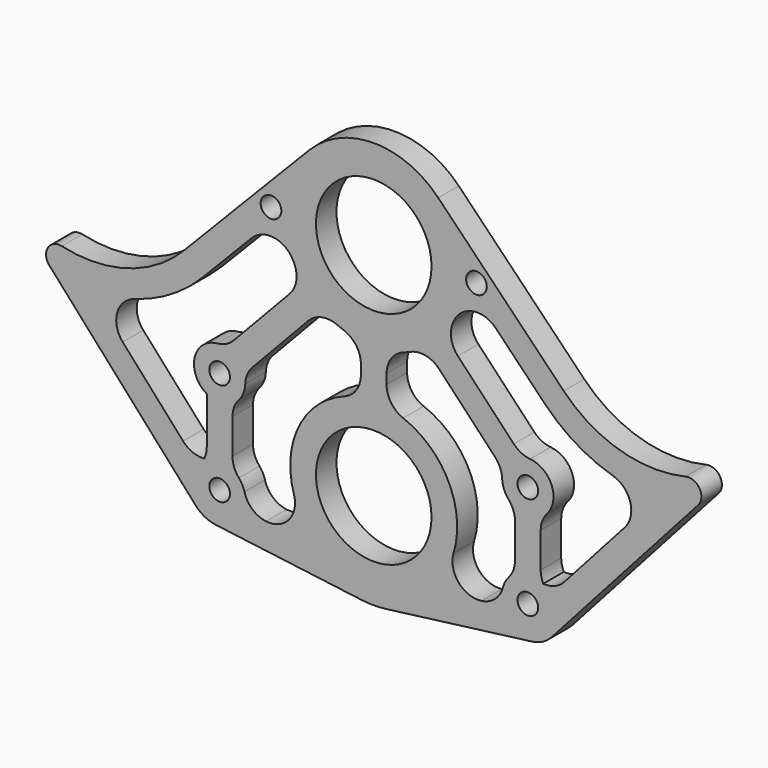
from build123d import *

# Parameters (mm, degrees)
F0_R        = 2.5527
F0_R_2      = 14.2875
F1_DEPTH    = 6.35
F3_DEPTH    = 25.4
F4_T1_DEPTH = 6.35


# Not quite as in the source:
# - a fillet or chamfer that OpenCascade refuses, or shapes differently, is made with other operations: its cross-section is extruded or revolved along the edge and cut away or added


with BuildPart() as f1:
    # F0 (on Front) → F1 (new body)
    with BuildSketch(Plane.XZ):
        with BuildLine():
            ThreePointArc((-3.0331353108, -25.2060360773), (0, -25.4), (3.0331353108, -25.2060360773))
            Line((3.0331353108, -25.2060360773), (39.1110451036, -20.5728453591))
            ThreePointArc((39.1110451036, -20.5728453591), (41.7972497423, -19.7238344651), (44.0177169487, -17.9900408661))
            Line((44.0177169487, -17.9900408661), (80.2059498117, 22.4920129361))
            ThreePointArc((80.2059498117, 22.4920129361), (80.5691803237, 26.2285207166), (77.1152341344, 27.6994668475))
            ThreePointArc((77.1152341344, 27.6994668475), (60.8820938076, 28.1479627769), (46.9763621139, 36.5352519414))
            Line((46.9763621139, 36.5352519414), (15.9477554983, 68.5021550209))
            ThreePointArc((15.9477554983, 68.5021550209), (0, 75.2475), (-15.9477554983, 68.5021550209))
            Line((-15.9477554983, 68.5021550209), (-46.9763621139, 36.5352519414))
            ThreePointArc((-46.9763621139, 36.5352519414), (-60.8820938076, 28.1479627769), (-77.1152341344, 27.6994668475))
            ThreePointArc((-77.1152341344, 27.6994668475), (-80.5691803237, 26.2285207166), (-80.2059498117, 22.4920129361))
            Line((-80.2059498117, 22.4920129361), (-44.0177169487, -17.9900408661))
            ThreePointArc((-44.0177169487, -17.9900408661), (-41.7972497423, -19.7238344651), (-39.1110451036, -20.5728453591))
            Line((-39.1110451036, -20.5728453591), (-3.0331353108, -25.2060360773))
        make_face()
        with Locations((-38.1, -12.7)):
            Circle(F0_R, mode=Mode.SUBTRACT)
        with Locations((0, -1.5875)):
            Circle(F0_R_2, mode=Mode.SUBTRACT)
        with Locations((-38.1, 12.7)):
            Circle(F0_R, mode=Mode.SUBTRACT)
        with Locations((38.1, -12.7)):
            Circle(F0_R, mode=Mode.SUBTRACT)
        with Locations((38.1, 12.7)):
            Circle(F0_R, mode=Mode.SUBTRACT)
        with Locations((-25.4, 53.0225)):
            Circle(F0_R, mode=Mode.SUBTRACT)
        with Locations((0, 53.0225)):
            Circle(F0_R_2, mode=Mode.SUBTRACT)
        with Locations((25.4, 53.0225)):
            Circle(F0_R, mode=Mode.SUBTRACT)
    extrude(amount=F1_DEPTH)

    # F2 (on face) → F3 (cut)
    with BuildSketch(Plane.XZ.offset(6.35)):
        with BuildLine():
            ThreePointArc((-43.3811914248, -9.1741643352), (-42.441704222, -8.0661997833), (-41.275, -7.200738686))
            Line((-41.275, -7.200738686), (-41.275, 7.200738686))
            ThreePointArc((-41.275, 7.200738686), (-44.0004697722, 15.046690535), (-36.6309164423, 18.8777255929))
            Line((-36.6309164423, 18.8777255929), (-17.4151480361, 39.2144138227))
            ThreePointArc((-17.4151480361, 39.2144138227), (-20.0010259245, 43.331804103), (-21.6296875, 47.9129752029))
            ThreePointArc((-21.6296875, 47.9129752029), (-24.6257359251, 46.7198802953), (-27.8214787465, 47.1523261797))
            Line((-27.8214787465, 47.1523261797), (-42.4198605429, 32.112493364))
            ThreePointArc((-42.4198605429, 32.112493364), (-54.9895844041, 23.5171709652), (-69.9173374643, 20.510559308))
            Line((-69.9173374643, 20.510559308), (-43.3811914248, -9.1741643352))
        make_face()
        with BuildLine():
            Line((-34.925, 7.200738686), (-34.925, -7.200738686))
            ThreePointArc((-34.925, -7.200738686), (-32.0996562634, -10.6219299715), (-32.2039292281, -15.0577212415))
            Line((-32.2039292281, -15.0577212415), (-13.1332337576, -17.5068145995))
            ThreePointArc((-13.1332337576, -17.5068145995), (-19.9026130173, 3.870741597), (-3.175, 18.8043067186))
            Line((-3.175, 18.8043067186), (-3.175, 31.0254547439))
            ThreePointArc((-3.175, 31.0254547439), (-8.2134168725, 32.3708557972), (-12.799622514, 34.8532873451))
            Line((-12.799622514, 34.8532873451), (-32.0153909201, 14.5165991152))
            ThreePointArc((-32.0153909201, 14.5165991152), (-32.1995302278, 10.353309465), (-34.925, 7.200738686))
        make_face()
        with BuildLine():
            Line((41.275, 7.200738686), (41.275, -7.200738686))
            ThreePointArc((41.275, -7.200738686), (42.441704222, -8.0661997833), (43.3811914248, -9.1741643352))
            Line((43.3811914248, -9.1741643352), (69.9173374643, 20.510559308))
            ThreePointArc((69.9173374643, 20.510559308), (54.9895844041, 23.5171709652), (42.4198605429, 32.112493364))
            Line((42.4198605429, 32.112493364), (27.8214787465, 47.1523261797))
            ThreePointArc((27.8214787465, 47.1523261797), (24.6257359251, 46.7198802953), (21.6296875, 47.9129752029))
            ThreePointArc((21.6296875, 47.9129752029), (20.0010259245, 43.331804103), (17.4151480361, 39.2144138227))
            Line((17.4151480361, 39.2144138227), (36.6309164423, 18.8777255929))
            ThreePointArc((36.6309164423, 18.8777255929), (44.0004697722, 15.046690535), (41.275, 7.200738686))
        make_face()
        with BuildLine():
            Line((13.1332337576, -17.5068145995), (32.2039292281, -15.0577212415))
            ThreePointArc((32.2039292281, -15.0577212415), (32.0996562634, -10.6219299715), (34.925, -7.200738686))
            Line((34.925, -7.200738686), (34.925, 7.200738686))
            ThreePointArc((34.925, 7.200738686), (32.1995302278, 10.353309465), (32.0153909201, 14.5165991152))
            Line((32.0153909201, 14.5165991152), (12.799622514, 34.8532873451))
            ThreePointArc((12.799622514, 34.8532873451), (8.2134168725, 32.3708557972), (3.175, 31.0254547439))
            Line((3.175, 31.0254547439), (3.175, 18.8043067186))
            ThreePointArc((3.175, 18.8043067186), (19.9026130173, 3.870741597), (13.1332337576, -17.5068145995))
        make_face()
    extrude(amount=-F3_DEPTH, mode=Mode.SUBTRACT)

    # F4: fillet of radius 6.35 on 31 edges, made by hand

    # F4_s2 → F4_t1 (join)
    with BuildSketch(Plane.XZ):
        with BuildLine():
            ThreePointArc((-25.4999328069, 46.6732863925), (-28.0274278752, 46.1917334318), (-30.1563671847, 44.7468313623))
            Line((-30.1563671847, 44.7468313623), (-27.8214787465, 47.1523261797))
            ThreePointArc((-27.8214787465, 47.1523261797), (-26.6832571196, 46.8035168705), (-25.4999328069, 46.6732863925))
        make_face()
        with BuildLine():
            ThreePointArc((-19.9098958333, 43.1459280792), (-22.2094720123, 45.6940981456), (-25.49921875, 46.6732751938))
            ThreePointArc((-25.49921875, 46.6732751938), (-23.4626186853, 46.9752647936), (-21.6296875, 47.9129752029))
            ThreePointArc((-21.6296875, 47.9129752029), (-20.9061098832, 45.4802725735), (-19.9098958333, 43.1459280792))
        make_face()
        with BuildLine():
            ThreePointArc((-20.8104553969, 35.621046866), (-19.1395225651, 39.0861033883), (-19.775762937, 42.8800237117))
            ThreePointArc((-19.775762937, 42.8800237117), (-18.6855596309, 40.9891926291), (-17.4151480361, 39.2144138227))
            Line((-17.4151480361, 39.2144138227), (-20.8104553969, 35.621046866))
        make_face()
        with BuildLine():
            ThreePointArc((-3.175, 23.6632332814), (-4.3022626627, 20.0513757668), (-7.2838235294, 17.721884274))
            ThreePointArc((-7.2838235294, 17.721884274), (-5.2573431495, 18.3691216895), (-3.175, 18.8043067186))
            Line((-3.175, 18.8043067186), (-3.175, 23.6632332814))
        make_face()
        with BuildLine():
            ThreePointArc((-38.6770301176, 19.0237280336), (-36.4785224973, 19.6361610946), (-34.6385347131, 20.9863295896))
            Line((-34.6385347131, 20.9863295896), (-36.6309164423, 18.8777255929))
            ThreePointArc((-36.6309164423, 18.8777255929), (-37.6480387039, 19.0338954038), (-38.6770301176, 19.0237280336))
        make_face()
        with BuildLine():
            ThreePointArc((-42.8625, -8.4998697937), (-41.6851188985, -6.5448036176), (-41.275, -4.2997395874))
            Line((-41.275, -4.2997395874), (-41.275, -7.200738686))
            ThreePointArc((-41.275, -7.200738686), (-42.1215559142, -7.7857769659), (-42.8625, -8.4998697937))
        make_face()
        with BuildLine():
            ThreePointArc((-47.1299420033, -4.9806154768), (-43.9553595951, -6.9040823934), (-40.2478842222, -6.724291392))
            ThreePointArc((-40.2478842222, -6.724291392), (-42.0112990938, -7.6975766474), (-43.3811914248, -9.1741643352))
            Line((-43.3811914248, -9.1741643352), (-47.1299420033, -4.9806154768))
        make_face()
        with BuildLine():
            ThreePointArc((-62.0621747984, 11.7233626833), (-63.433674019, 17.6998895462), (-59.1117617466, 22.0497122742))
            ThreePointArc((-59.1117617466, 22.0497122742), (-64.4593340972, 20.8924970257), (-69.9173374643, 20.510559308))
            Line((-69.9173374643, 20.510559308), (-62.0621747984, 11.7233626833))
        make_face()
        with BuildLine():
            ThreePointArc((-34.925, -4.2997395874), (-34.5148811015, -6.5448036176), (-33.3375, -8.4998697937))
            ThreePointArc((-33.3375, -8.4998697937), (-34.0784440858, -7.7857769659), (-34.925, -7.200738686))
            Line((-34.925, -7.200738686), (-34.925, -4.2997395874))
        make_face()
        with BuildLine():
            ThreePointArc((-33.3375, 8.4998697937), (-34.5148811015, 6.5448036176), (-34.925, 4.2997395874))
            Line((-34.925, 4.2997395874), (-34.925, 7.200738686))
            ThreePointArc((-34.925, 7.200738686), (-34.0784440858, 7.7857769659), (-33.3375, 8.4998697937))
        make_face()
        with BuildLine():
            ThreePointArc((-30.0230091909, 16.625203112), (-31.2668035127, 14.7117022115), (-31.7537418344, 12.4820383172))
            ThreePointArc((-31.7537418344, 12.4820383172), (-31.8018673776, 13.5099539932), (-32.0153909201, 14.5165991152))
            Line((-32.0153909201, 14.5165991152), (-30.0230091909, 16.625203112))
        make_face()
        with BuildLine():
            ThreePointArc((-31.9580280848, -11.087957509), (-30.0075511004, -14.2460167198), (-26.6248922524, -15.7741913054))
            Line((-26.6248922524, -15.7741913054), (-32.2039292281, -15.0577212415))
            ThreePointArc((-32.2039292281, -15.0577212415), (-31.762147528, -13.092588898), (-31.9580280848, -11.087957509))
        make_face()
        with BuildLine():
            ThreePointArc((3.175, 23.6632332814), (4.3022626627, 20.0513757668), (7.2838235294, 17.721884274))
            ThreePointArc((7.2838235294, 17.721884274), (5.2573431495, 18.3691216895), (3.175, 18.8043067186))
            Line((3.175, 18.8043067186), (3.175, 23.6632332814))
        make_face()
        with BuildLine():
            ThreePointArc((-26.6174183984, -15.7751511113), (-20.9556247606, -13.572152955), (-19.7359747119, -7.620551336))
            ThreePointArc((-19.7359747119, -7.620551336), (-17.161898691, -13.0494212861), (-13.1332337576, -17.5068145995))
            Line((-13.1332337576, -17.5068145995), (-26.6174183984, -15.7751511113))
        make_face()
        with BuildLine():
            ThreePointArc((26.6248922524, -15.7741913054), (30.0075511004, -14.2460167198), (31.9580280848, -11.087957509))
            ThreePointArc((31.9580280848, -11.087957509), (31.762147528, -13.092588898), (32.2039292281, -15.0577212415))
            Line((32.2039292281, -15.0577212415), (26.6248922524, -15.7741913054))
        make_face()
        with BuildLine():
            ThreePointArc((33.3375, -8.4998697937), (34.5148811015, -6.5448036176), (34.925, -4.2997395874))
            Line((34.925, -4.2997395874), (34.925, -7.200738686))
            ThreePointArc((34.925, -7.200738686), (34.0784440858, -7.7857769659), (33.3375, -8.4998697937))
        make_face()
        with BuildLine():
            ThreePointArc((26.6174183984, -15.7751511113), (20.9556247606, -13.572152955), (19.7359747119, -7.620551336))
            ThreePointArc((19.7359747119, -7.620551336), (17.161898691, -13.0494212861), (13.1332337576, -17.5068145995))
            Line((13.1332337576, -17.5068145995), (26.6174183984, -15.7751511113))
        make_face()
        with BuildLine():
            ThreePointArc((34.6385347131, 20.9863295896), (36.4785224973, 19.6361610946), (38.6770301176, 19.0237280336))
            ThreePointArc((38.6770301176, 19.0237280336), (37.6480387039, 19.0338954038), (36.6309164423, 18.8777255929))
            Line((36.6309164423, 18.8777255929), (34.6385347131, 20.9863295896))
        make_face()
        with BuildLine():
            ThreePointArc((42.8625, 8.4998697937), (41.6851188985, 6.5448036176), (41.275, 4.2997395874))
            Line((41.275, 4.2997395874), (41.275, 7.200738686))
            ThreePointArc((41.275, 7.200738686), (42.1215559142, 7.7857769659), (42.8625, 8.4998697937))
        make_face()
        with BuildLine():
            ThreePointArc((19.775762937, 42.8800237117), (19.1395225651, 39.0861033883), (20.8104553969, 35.621046866))
            Line((20.8104553969, 35.621046866), (17.4151480361, 39.2144138227))
            ThreePointArc((17.4151480361, 39.2144138227), (18.6855596309, 40.9891926291), (19.775762937, 42.8800237117))
        make_face()
        with BuildLine():
            ThreePointArc((-9.0062033853, 32.7040619305), (-12.8300676147, 33.1244136714), (-16.1949298747, 31.2599203883))
            Line((-16.1949298747, 31.2599203883), (-12.799622514, 34.8532873451))
            ThreePointArc((-12.799622514, 34.8532873451), (-10.955742935, 33.685428822), (-9.0062033853, 32.7040619305))
        make_face()
        with BuildLine():
            ThreePointArc((7.4083333333, 32.0685690508), (4.3402467111, 29.7479058461), (3.175, 26.0817316368))
            Line((3.175, 26.0817316368), (3.175, 31.0254547439))
            ThreePointArc((3.175, 31.0254547439), (5.317307399, 31.442952576), (7.4083333333, 32.0685690508))
        make_face()
        with BuildLine():
            ThreePointArc((-3.175, 26.0817316368), (-4.3402467111, 29.7479058461), (-7.4083333333, 32.0685690508))
            ThreePointArc((-7.4083333333, 32.0685690508), (-5.317307399, 31.442952576), (-3.175, 31.0254547439))
            Line((-3.175, 31.0254547439), (-3.175, 26.0817316368))
        make_face()
        with BuildLine():
            ThreePointArc((16.1949298747, 31.2599203883), (12.8300676147, 33.1244136714), (9.0062033853, 32.7040619305))
            ThreePointArc((9.0062033853, 32.7040619305), (10.955742935, 33.685428822), (12.799622514, 34.8532873451))
            Line((12.799622514, 34.8532873451), (16.1949298747, 31.2599203883))
        make_face()
        with BuildLine():
            ThreePointArc((31.7537418344, 12.4820383172), (31.2668035127, 14.7117022115), (30.0230091909, 16.625203112))
            Line((30.0230091909, 16.625203112), (32.0153909201, 14.5165991152))
            ThreePointArc((32.0153909201, 14.5165991152), (31.8018673776, 13.5099539932), (31.7537418344, 12.4820383172))
        make_face()
        with BuildLine():
            ThreePointArc((34.925, 4.2997395874), (34.5148811015, 6.5448036176), (33.3375, 8.4998697937))
            ThreePointArc((33.3375, 8.4998697937), (34.0784440858, 7.7857769659), (34.925, 7.200738686))
            Line((34.925, 7.200738686), (34.925, 4.2997395874))
        make_face()
        with BuildLine():
            ThreePointArc((62.0621747984, 11.7233626833), (63.433674019, 17.6998895462), (59.1117617466, 22.0497122742))
            ThreePointArc((59.1117617466, 22.0497122742), (64.4593340972, 20.8924970257), (69.9173374643, 20.510559308))
            Line((69.9173374643, 20.510559308), (62.0621747984, 11.7233626833))
        make_face()
        with BuildLine():
            ThreePointArc((25.49921875, 46.6732751938), (22.2094720123, 45.6940981456), (19.9098958333, 43.1459280792))
            ThreePointArc((19.9098958333, 43.1459280792), (20.9061098832, 45.4802725735), (21.6296875, 47.9129752029))
            ThreePointArc((21.6296875, 47.9129752029), (23.4626186853, 46.9752647936), (25.49921875, 46.6732751938))
        make_face()
        with BuildLine():
            ThreePointArc((30.1563671847, 44.7468313623), (28.0274278752, 46.1917334318), (25.4999328069, 46.6732863925))
            ThreePointArc((25.4999328069, 46.6732863925), (26.6832571196, 46.8035168705), (27.8214787465, 47.1523261797))
            Line((27.8214787465, 47.1523261797), (30.1563671847, 44.7468313623))
        make_face()
        with BuildLine():
            ThreePointArc((41.275, -4.2997395874), (41.6851188985, -6.5448036176), (42.8625, -8.4998697937))
            ThreePointArc((42.8625, -8.4998697937), (42.1215559142, -7.7857769659), (41.275, -7.200738686))
            Line((41.275, -7.200738686), (41.275, -4.2997395874))
        make_face()
        with BuildLine():
            ThreePointArc((40.2478842222, -6.724291392), (43.9553595951, -6.9040823934), (47.1299420033, -4.9806154768))
            Line((47.1299420033, -4.9806154768), (43.3811914248, -9.1741643352))
            ThreePointArc((43.3811914248, -9.1741643352), (42.0112990938, -7.6975766474), (40.2478842222, -6.724291392))
        make_face()
    extrude(amount=F4_T1_DEPTH)


solid = f1.part
